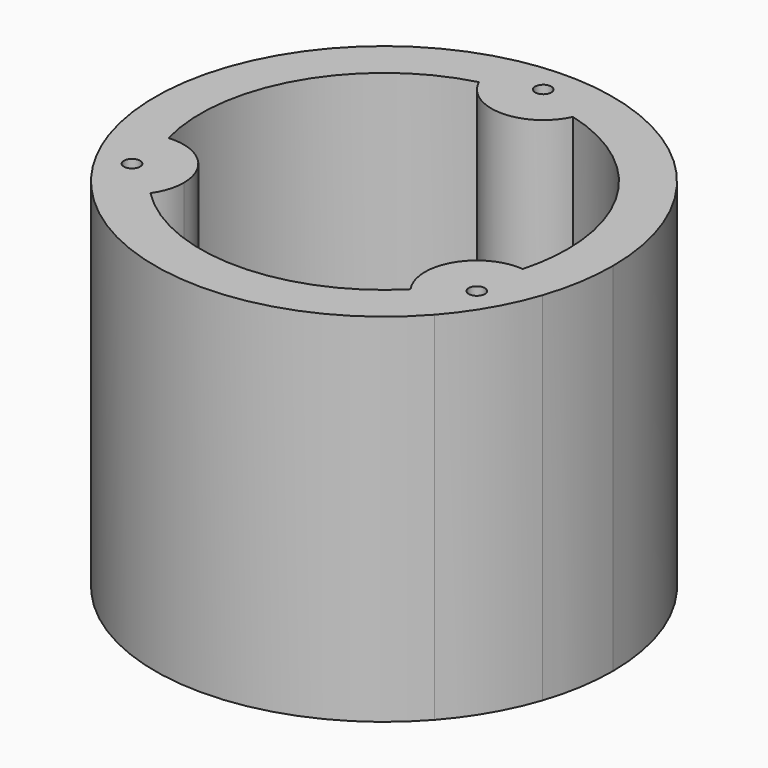
from build123d import *

# Parameters (mm, degrees)
F0_R     = 1.5875
F1_DEPTH = 70


with BuildPart() as f1:
    # F0 (on Top) → F1 (new body)
    with BuildSketch(Plane.XY):
        with BuildLine():
            ThreePointArc((42.5527261375, -14.32743865), (44.3092958846, -7.2592215983), (44.9, 0))
            ThreePointArc((44.9, 0), (34.7433650607, 28.4413182581), (8.8684372267, 44.0154611603))
            ThreePointArc((8.8684372267, 44.0154611603), (9.8318086389, 41.6194720159), (10.16, 39.058))
            ThreePointArc((10.16, 39.058), (9.9243037361, 36.8822713051), (9.2281505209, 34.807489682))
            ThreePointArc((9.2281505209, 34.807489682), (28.53967239, 21.9592167408), (36.01, 0))
            ThreePointArc((36.01, 0), (35.6956896759, -4.7474033498), (34.758245567, -9.4119320599))
            ThreePointArc((34.758245567, -9.4119320599), (39.2448159004, -10.9351892811), (42.5527261375, -14.32743865))
        make_face()
        with BuildLine():
            ThreePointArc((10.16, 39.058), (9.8318086389, 41.6194720159), (8.8684372267, 44.0154611603))
            ThreePointArc((8.8684372267, 44.0154611603), (0, 44.9), (-8.8684372267, 44.0154611603))
            ThreePointArc((-8.8684372267, 44.0154611603), (-10.1522562376, 39.4546021771), (-9.2281505209, 34.807489682))
            ThreePointArc((-9.2281505209, 34.807489682), (0, 36.01), (9.2281505209, 34.807489682))
            ThreePointArc((9.2281505209, 34.807489682), (9.9243037361, 36.8822713051), (10.16, 39.058))
        make_face()
        with Locations((0, 39.058)):
            Circle(F0_R, mode=Mode.SUBTRACT)
        with BuildLine():
            ThreePointArc((33.6842889108, -29.6880225103), (38.8845406299, -22.45), (42.5527261375, -14.32743865))
            ThreePointArc((42.5527261375, -14.32743865), (39.2448159004, -10.9351892811), (34.758245567, -9.4119320599))
            ThreePointArc((34.758245567, -9.4119320599), (31.1855747903, -18.005), (25.5300950461, -25.3955576221))
            ThreePointArc((25.5300950461, -25.3955576221), (29.0925596628, -28.519412896), (33.6842889108, -29.6880225103))
        make_face()
        with Locations((33.825220221, -19.529)):
            Circle(F0_R, mode=Mode.SUBTRACT)
        with BuildLine():
            ThreePointArc((-9.2281505209, 34.807489682), (-10.1522562376, 39.4546021771), (-8.8684372267, 44.0154611603))
            ThreePointArc((-8.8684372267, 44.0154611603), (-38.8845406299, 22.45), (-42.5527261375, -14.32743865))
            ThreePointArc((-42.5527261375, -14.32743865), (-39.2448159004, -10.9351892811), (-34.758245567, -9.4119320599))
            ThreePointArc((-34.758245567, -9.4119320599), (-31.1855747903, 18.005), (-9.2281505209, 34.807489682))
        make_face()
        with BuildLine():
            ThreePointArc((-33.6842889108, -29.6880225103), (0, -44.9), (33.6842889108, -29.6880225103))
            ThreePointArc((33.6842889108, -29.6880225103), (29.0925596628, -28.519412896), (25.5300950461, -25.3955576221))
            ThreePointArc((25.5300950461, -25.3955576221), (0, -36.01), (-25.5300950461, -25.3955576221))
            ThreePointArc((-25.5300950461, -25.3955576221), (-29.0925596628, -28.519412896), (-33.6842889108, -29.6880225103))
        make_face()
        with BuildLine():
            ThreePointArc((25.5300950461, -25.3955576221), (31.1855747903, -18.005), (34.758245567, -9.4119320599))
            ThreePointArc((34.758245567, -9.4119320599), (25.0264021186, -14.449), (25.5300950461, -25.3955576221))
        make_face()
        with BuildLine():
            ThreePointArc((-34.758245567, -9.4119320599), (-39.2448159004, -10.9351892811), (-42.5527261375, -14.32743865))
            ThreePointArc((-42.5527261375, -14.32743865), (-38.8845406299, -22.45), (-33.6842889108, -29.6880225103))
            ThreePointArc((-33.6842889108, -29.6880225103), (-29.0925596628, -28.519412896), (-25.5300950461, -25.3955576221))
            ThreePointArc((-25.5300950461, -25.3955576221), (-31.1855747903, -18.005), (-34.758245567, -9.4119320599))
        make_face()
        with Locations((-33.825220221, -19.529)):
            Circle(F0_R, mode=Mode.SUBTRACT)
        with BuildLine():
            ThreePointArc((9.2281505209, 34.807489682), (0, 36.01), (-9.2281505209, 34.807489682))
            ThreePointArc((-9.2281505209, 34.807489682), (0, 28.898), (9.2281505209, 34.807489682))
        make_face()
        with BuildLine():
            ThreePointArc((-23.665220221, -19.529), (-26.9788320315, -12.0221651971), (-34.758245567, -9.4119320599))
            ThreePointArc((-34.758245567, -9.4119320599), (-31.1855747903, -18.005), (-25.5300950461, -25.3955576221))
            ThreePointArc((-25.5300950461, -25.3955576221), (-24.1426567232, -22.6069155465), (-23.665220221, -19.529))
        make_face()
    extrude(amount=F1_DEPTH)


solid = f1.part
